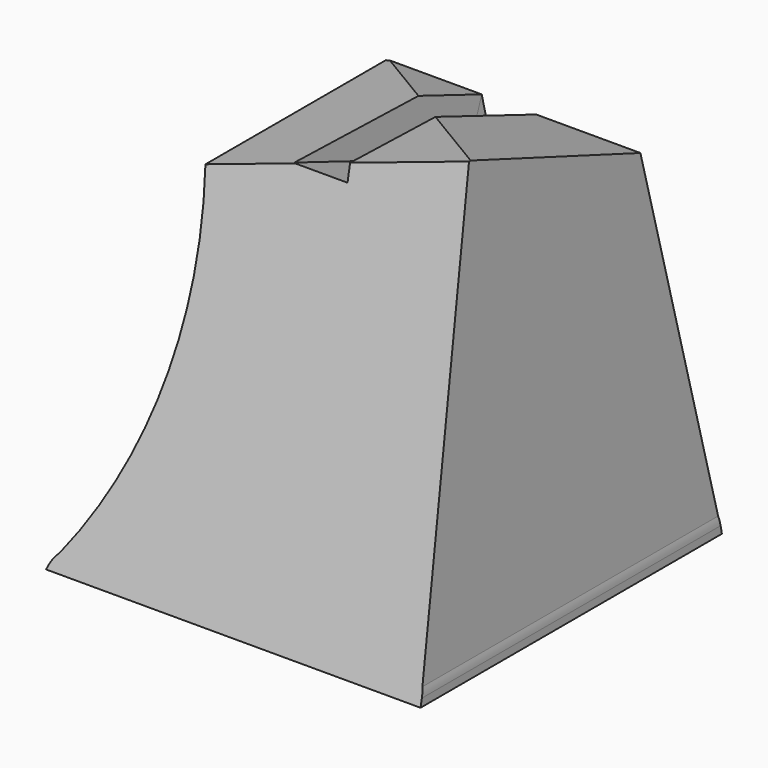
from build123d import *

# Parameters (mm, degrees)
F0_W         = 45
F0_H         = 45
F1_DEPTH     = 2
F3_DEPTH     = 45
F5_DEPTH     = 50
F7_DEPTH     = 52.4
F9_DEPTH     = 6.25
F10_T1_DEPTH = 62.3121019707
F11_T1_DEPTH = 49.4942070429


# Not quite as in the source:
# - a fillet or chamfer that OpenCascade refuses, or shapes differently, is made with other operations: its cross-section is extruded or revolved along the edge and cut away or added


with BuildPart() as f1:
    # F0 (on Top) → F1 (new body)
    with BuildSketch(Plane.XY):
        with Locations((-22.5, 22.5)):
            Rectangle(F0_W, F0_H)
    extrude(amount=F1_DEPTH)

    # F2 (on Front) → F3 (join)
    with BuildSketch(Plane.XZ):
        with BuildLine():
            Line((-45, 0), (0, 0))
            Line((0, 0), (-3, 52))
            Line((-3, 52), (-32.9244207251, 42.7682981249))
            ThreePointArc((-32.9244207251, 42.7682981249), (-34.5043559539, 20.1254790506), (-45, 0))
        make_face()
    extrude(amount=-F3_DEPTH)

    # F4 (on Right) → F5 (cut)
    with BuildSketch(Plane.YZ):
        Polygon((0, 0), (12.5, 59.1310895979), (0, 59.1310895979), align=None)
        Polygon((45, 0), (45, 59.1310895979), (32.5, 59.1310895979), align=None)
    extrude(amount=-F5_DEPTH, mode=Mode.SUBTRACT)

    # F6 (on Right) → F7 (cut)
    with BuildSketch(Plane.YZ):
        Polygon((37.7679802477, 54.4090420008), (10.9807690606, 52.094515413), (37.7679802477, 42.2525405884), align=None)
    extrude(amount=-F7_DEPTH, mode=Mode.SUBTRACT)

    # F8 (on face) → F9 (cut)
    with BuildSketch(Plane(origin=(0, 18.1697536282, 49.4531876304), x_dir=(1, 0, 0), z_dir=(0, 0.3448722583, 0.9386496287))):
        Polygon((-14.9190827221, 18.9156103945), (-13.4748989156, 42.5651032579), (-19.9628132083, 42.9612952953), (-21.4311909427, 18.9156103945), align=None)
        Polygon((-15.8245932316, 4.0872594346), (-14.9190827221, 18.9156103945), (-21.4311909427, 18.9156103945), (-21.9993973802, 9.6108432114), align=None)
        Polygon((-17.0844251269, -16.5433453977), (-15.8245932316, 4.0872594346), (-21.9993973802, 9.6108432114), (-23.5723394196, -16.1471533603), align=None)
    extrude(amount=-F9_DEPTH, mode=Mode.SUBTRACT)

    # F10: fillet of radius 5 on 1 edges, made by hand

    # F10_s2 → F10_t1 (cut)
    with BuildSketch(Plane.XZ.offset(-53.6560509853)):
        with BuildLine():
            ThreePointArc((-45, -1.6315361684), (-44.5926166392, 0.3452977662), (-43.436851038, 2))
            Line((-43.436851038, 2), (-45, 2))
            Line((-45, 2), (-45, -1.6315361684))
        make_face()
    extrude(amount=F10_T1_DEPTH, mode=Mode.SUBTRACT)

    # F11: fillet of radius 5 on 1 edges, made by hand

    # F11_s2 → F11_t1 (cut)
    with BuildSketch(Plane.XZ.offset(-47.2471035215)):
        with BuildLine():
            ThreePointArc((0, 0.9320428172), (-0.0289298475, 1.4691289727), (-0.1153846154, 2))
            Line((-0.1153846154, 2), (0, 2))
            Line((0, 2), (0, 0.9320428172))
        make_face()
    extrude(amount=F11_T1_DEPTH, mode=Mode.SUBTRACT)


solid = f1.part
